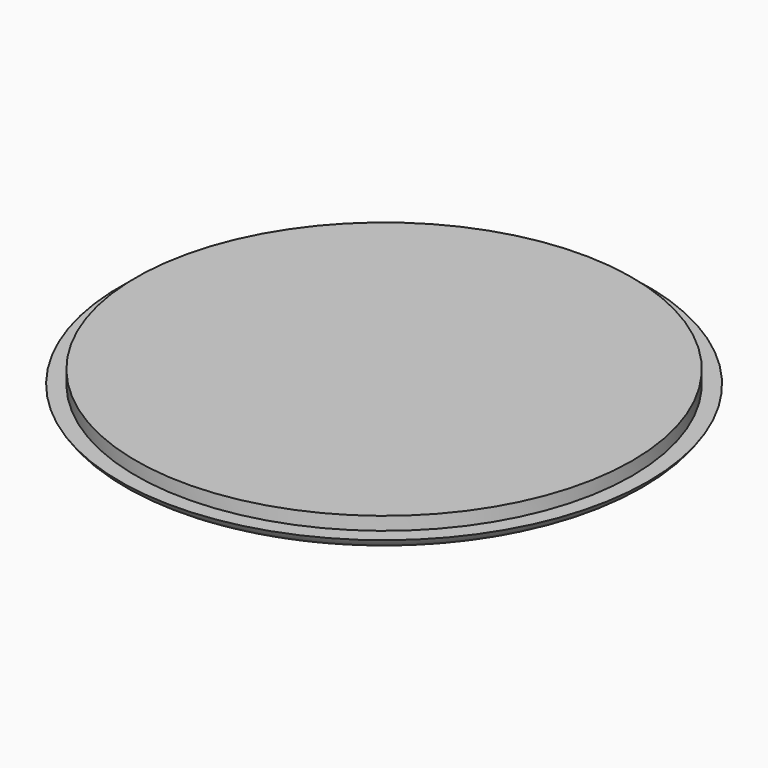
from build123d import *

# Parameters (mm, degrees)
F0_R         = 50.8
F1_DEPTH     = 2.54
F2_R         = 47.752
F3_DEPTH     = 2.54
F5_TEXT_SIZE = 35.2777777778
F6_DEPTH     = 2.54


# Not quite as in the source:
# - a fillet or chamfer that OpenCascade refuses, or shapes differently, is made with other operations: its cross-section is extruded or revolved along the edge and cut away or added
# - Text() gives the source's letters only with a copy of the font that has no kerning and outlines rounded to 1/6400 em; it was checked with that copy


with BuildPart() as f1:
    # F0 (on Top) → F1 (new body)
    with BuildSketch(Plane.XY):
        Circle(F0_R)
    extrude(amount=F1_DEPTH)

    # F2 (on face) → F3 (join)
    with BuildSketch(Plane.XY.offset(2.54)):
        Circle(F2_R)
    extrude(amount=F3_DEPTH)

    # F4: fillet of radius 5.08 on 1 edges, made by hand

    # F4_s1 → F4_t2 (revolve, cut)
    with BuildSketch(Plane.XZ):
        with BuildLine():
            ThreePointArc((50.8, 2.54), (48.9405909488, 0.6805909488), (46.4005909488, 0))
            Line((46.4005909488, 0), (50.8, 0))
            Line((50.8, 0), (50.8, 2.54))
        make_face()
    revolve(axis=Axis((0, 0, 0), (0, 0, 1)), mode=Mode.SUBTRACT)

    # F5 (on face) → F6 (cut)
    with BuildSketch(Plane(origin=(0, 0, 0), x_dir=(1, 0, 0), z_dir=(0, 0, -1))):
        with Locations((-40.4206163194, -10.6814567984)):
            Text('KAO', F5_TEXT_SIZE, font='Tinos', font_style=FontStyle.BOLD, text_align=(TextAlign.LEFT, TextAlign.BOTTOM))
        with BuildLine():
            Line((22.5025620311, 1.8012444489), (21.4558970183, 1.8012444489))
            Line((21.4558970183, 1.8012444489), (21.4558970183, -0.6491758395))
            Line((21.4558970183, -0.6491758395), (22.5025620311, -0.6491758395))
            Line((22.5025620311, -0.6491758395), (22.5025620311, -0.5009419216))
            ThreePointArc((22.5025620311, -0.5009419216), (22.5449927776, -0.3985050381), (22.6474296611, -0.3560742916))
            Line((22.6474296611, -0.3560742916), (30.1213353562, -0.3560742916))
            ThreePointArc((30.1213353562, -0.3560742916), (30.2237722398, -0.3985050381), (30.2662029862, -0.5009419216))
            Line((30.2662029862, -0.5009419216), (30.2662029862, -0.6491758395))
            Line((30.2662029862, -0.6491758395), (31.3128679991, -0.6491758395))
            Line((31.3128679991, -0.6491758395), (31.3128679991, 1.8012444489))
            Line((31.3128679991, 1.8012444489), (30.2662029862, 1.8012444489))
            Line((30.2662029862, 1.8012444489), (30.2662029862, 1.7177510454))
            ThreePointArc((30.2662029862, 1.7177510454), (30.2237722398, 1.6153141618), (30.1213353562, 1.5728834154))
            Line((30.1213353562, 1.5728834154), (22.6474296611, 1.5728834154))
            ThreePointArc((22.6474296611, 1.5728834154), (22.5449927776, 1.6153141618), (22.5025620311, 1.7177510454))
            Line((22.5025620311, 1.7177510454), (22.5025620311, 1.8012444489))
        make_face()
    extrude(amount=-F6_DEPTH, mode=Mode.SUBTRACT)


solid = f1.part
